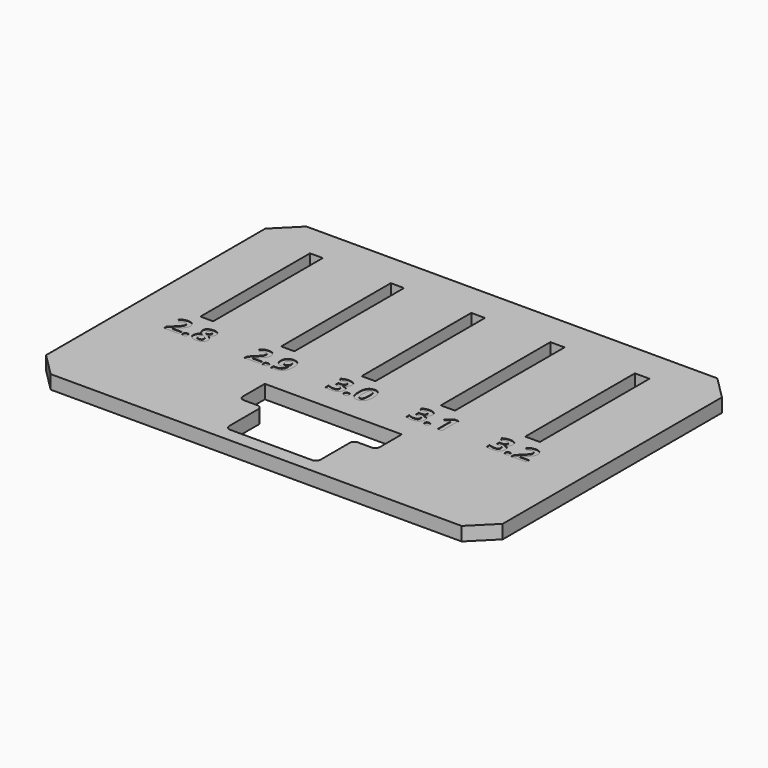
from build123d import *

# Parameters (mm, degrees)
F0_W         = 100
F0_H         = 70
F0_W_2       = 2.8
F0_H_2       = 30
F0_W_3       = 2.9
F0_W_4       = 3
F0_W_5       = 3.1
F0_W_6       = 3.2
F1_DEPTH     = 3
F2_TEXT_SIZE = 6.4706105375
F3_DEPTH     = 0.1
F4_SIZE      = 5


# Not quite as in the source:
# - Text() gives the source's letters only with a copy of the font that has no kerning and outlines rounded to 1/6400 em; it was checked with that copy


with BuildPart() as f1:
    # F0 (on Top) → F1 (new body)
    with BuildSketch(Plane.XY):
        Rectangle(F0_W, F0_H)
        with BuildLine():
            Line((-14.1631150595, -20.9241350167), (-14.1631150595, -14.9241350167))
            Line((-14.1631150595, -14.9241350167), (15.8368849405, -14.9241350167))
            Line((15.8368849405, -14.9241350167), (15.8368849405, -20.9241350167))
            ThreePointArc((15.8368849405, -20.9241350167), (15.5439917217, -21.6312417979), (14.8368849405, -21.9241350167))
            Line((14.8368849405, -21.9241350167), (11.8368849405, -21.9241350167))
            ThreePointArc((11.8368849405, -21.9241350167), (11.1297781593, -22.2170282355), (10.8368849405, -22.9241350167))
            Line((10.8368849405, -22.9241350167), (10.8368849405, -30.9241350167))
            ThreePointArc((10.8368849405, -30.9241350167), (10.5439917217, -31.6312417979), (9.8368849405, -31.9241350167))
            Line((9.8368849405, -31.9241350167), (-8.1631150595, -31.9241350167))
            ThreePointArc((-8.1631150595, -31.9241350167), (-8.8702218407, -31.6312417979), (-9.1631150595, -30.9241350167))
            Line((-9.1631150595, -30.9241350167), (-9.1631150595, -22.9241350167))
            ThreePointArc((-9.1631150595, -22.9241350167), (-9.4560082783, -22.2170282355), (-10.1631150595, -21.9241350167))
            Line((-10.1631150595, -21.9241350167), (-13.1631150595, -21.9241350167))
            ThreePointArc((-13.1631150595, -21.9241350167), (-13.8702218407, -21.6312417979), (-14.1631150595, -20.9241350167))
        make_face(mode=Mode.SUBTRACT)
        with Locations((-36.9171057329, 12.6378286374)):
            Rectangle(F0_W_2, F0_H_2, mode=Mode.SUBTRACT)
        with Locations((-19.1763875589, 12.6378286374)):
            Rectangle(F0_W_3, F0_H_2, mode=Mode.SUBTRACT)
        with Locations((-1.5, 12.6378286374)):
            Rectangle(F0_W_4, F0_H_2, mode=Mode.SUBTRACT)
        with Locations((15.8795573071, 12.6378286374)):
            Rectangle(F0_W_5, F0_H_2, mode=Mode.SUBTRACT)
        with Locations((34.4264879063, 12.6378286374)):
            Rectangle(F0_W_6, F0_H_2, mode=Mode.SUBTRACT)
    extrude(amount=F1_DEPTH)

    # F2 (on face) → F3 (cut)
    with BuildSketch(Plane.XY.offset(3)):
        with Locations((-40.7827587591, -9.5908074241)):
            Text('2.8     2.9     3.0     3.1     3.2', F2_TEXT_SIZE, font='Open Sans', font_style=FontStyle.BOLD, text_align=(TextAlign.LEFT, TextAlign.BOTTOM))
    extrude(amount=-F3_DEPTH, mode=Mode.SUBTRACT)

    # F4
    f4_edges = [f1.edges().sort_by_distance(p)[0] for p in [
        (-50, -35, 1.5),
        (50, -35, 1.5),
        (50, 35, 1.5),
        (-50, 35, 1.5),
    ]]
    chamfer(f4_edges, length=F4_SIZE)


solid = f1.part
